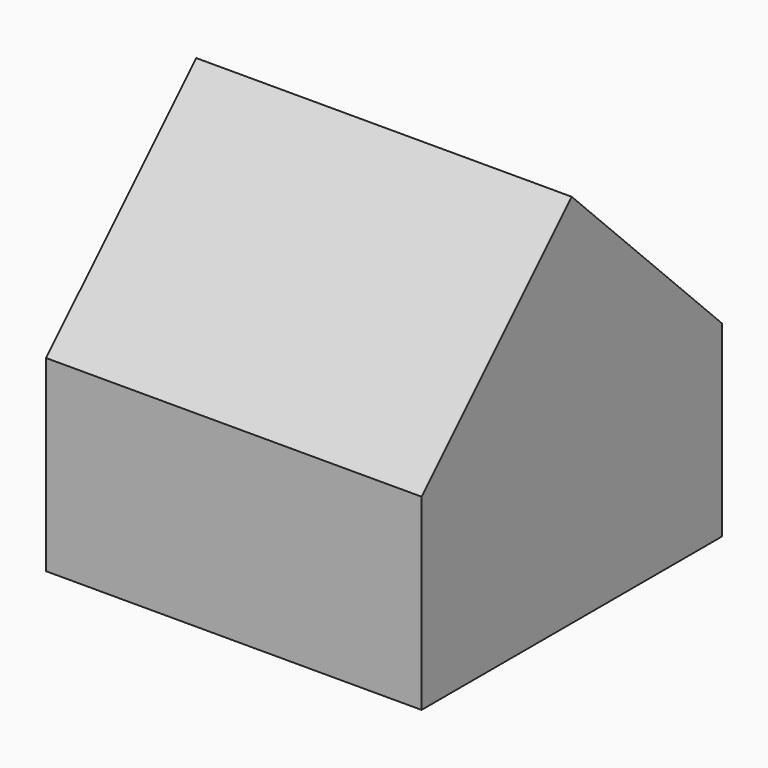
from build123d import *

# Parameters (mm, degrees)
F0_W     = 50
F0_H     = 50
F0_W_2   = 40
F0_H_2   = 40
F1_DEPTH = 25
F2_W     = 50
F2_H     = 50
F2_W_2   = 40
F2_H_2   = 40
F3_DEPTH = 25
F4_SIZE  = 24.99999


# Not quite as in the source:
# - a fillet or chamfer is up to 0.001 mm smaller than in the source, because OpenCascade refuses the exact size


with BuildPart() as f1:
    # F0 (on Top) → F1 (new body)
    with BuildSketch(Plane.XY):
        with Locations((25, 25)):
            Rectangle(F0_W, F0_H)
        with Locations((25, 25)):
            Rectangle(F0_W_2, F0_H_2, mode=Mode.SUBTRACT)
    extrude(amount=F1_DEPTH)

    # F2 (on face) → F3 (join)
    with BuildSketch(Plane.XY.offset(25)):
        with Locations((25, 25)):
            Rectangle(F2_W, F2_H)
        with Locations((25, 25)):
            Rectangle(F2_W_2, F2_H_2, mode=Mode.SUBTRACT)
        with Locations((25, 25)):
            Rectangle(F2_W_2, F2_H_2)
    extrude(amount=F3_DEPTH)

    # F4 (size 25 in the source; OpenCascade refuses exactly that, so slightly less here)
    f4_edges = [f1.edges().sort_by_distance(p)[0] for p in [
        (25, 0, 50),
        (25, 50, 50),
    ]]
    chamfer(f4_edges, length=F4_SIZE)


solid = f1.part
